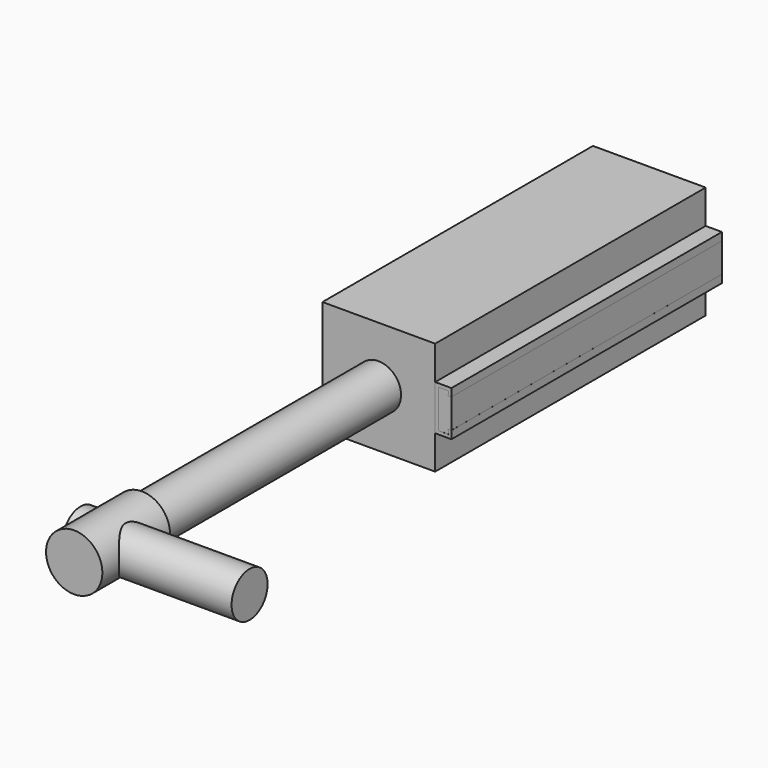
from build123d import *

# Parameters (mm, degrees)
F0_W              = 100
F0_H              = 300
F1_DEPTH          = 50
F2_R              = 20
F3_DEPTH          = 250
F4_DEPTH          = 300
F5_R              = 25
F6_DEPTH          = 37.5
F8_R              = 20
F9_DEPTH          = 50
F11_DEPTH         = 75
F18_D             = 3.5
F18_DEPTH         = 18
F18_CSINK_D       = 8.96
F18_CSINK_ANGLE   = 90
F18_TIP           = 1.0515060833
F18_2_D           = 3.5
F18_2_DEPTH       = 18
F18_2_CSINK_D     = 8.96
F18_2_CSINK_ANGLE = 90
F18_2_TIP         = 1.0515060833


# Not quite as in the source:
# - a feature of the source that left no trace in its solid (it failed there, or was rolled back) is left out


with BuildPart() as f1:
    # F0 (on Top) → F1 (new body, symmetric)
    with BuildSketch(Plane.XY):
        with Locations((0.3009543288, 62.5117615233)):
            Rectangle(F0_W, F0_H)
    extrude(amount=F1_DEPTH, both=True)

    # F2 (on face) → F3 (cut)
    with BuildSketch(Plane.XZ.offset(87.4882384767)):
        Circle(F2_R)
    extrude(amount=-F3_DEPTH, mode=Mode.SUBTRACT)

    # F18
    with Locations(Plane.YZ.offset(53.3009543288)):
        with Locations((162.5128239393, 0), (0, 0)):
            CounterSinkHole(F18_D / 2, F18_CSINK_D / 2, depth=F18_DEPTH, counter_sink_angle=F18_CSINK_ANGLE)
            with Locations((0, 0, -(F18_DEPTH + F18_TIP / 2))):  # 118° drill point
                Cone(0, F18_D / 2, F18_TIP, mode=Mode.SUBTRACT)


with BuildPart() as f4:
    # F2 (on face) → F4 (new body)
    with BuildSketch(Plane.XZ.offset(87.4882384767)):
        Circle(F2_R)
    extrude(amount=F4_DEPTH)

    # F5 (on face) → F6 (join, symmetric)
    with BuildSketch(Plane.XZ.offset(387.4882384767)):
        Circle(F5_R)
    extrude(amount=F6_DEPTH, both=True)


with BuildPart() as f9:
    # F8 (on Right) → F9 (new body, symmetric)
    with BuildSketch(Plane.YZ):
        with Locations((-386.7093552819, 0)):
            Circle(F8_R)
    extrude(amount=F9_DEPTH, both=True)


with BuildPart() as f4_1:
    add(f4.part)

    # F10: cut F9
    add(f9.part, mode=Mode.SUBTRACT)


with BuildPart() as f11:
    # F8 (on Right) → F11 (new body, symmetric)
    with BuildSketch(Plane.YZ):
        with Locations((-386.7093552819, 0)):
            Circle(F8_R)
    extrude(amount=F11_DEPTH, both=True)


with BuildPart() as f12_1:
    # F12: copy of F11
    add(f11.part.moved(Location((50, 0, 0))))


with BuildPart() as f16:
    # F16: sweep along a path in F15
    with BuildLine(Plane.YZ.offset(50.3009543288)) as f16_path:
        Line((-87.4882384767, 0), (212.5117615233, 0))
    # F14 (on face) → F16 (sweep)
    with BuildSketch(Plane(origin=(0, 212.5117615233, 0), x_dir=(-1, 0, 0), z_dir=(0, 1, 0))):
        Polygon((-50.3009543288, -20), (-50.3009543288, 20), (-64.7470878231, 20), (-64.7470878231, 13), (-61.7470878231, 13), (-62.3009543288, 16.9614684012), (-53.3009543288, 16.9614684012), (-53.3009543288, -17), (-62.3009543288, -17), (-61.7470878231, -13), (-64.7470878231, -13), (-64.7470878231, -20), align=None)
    sweep(path=f16_path.line)

    # F18#2
    with Locations(Plane.YZ.offset(53.3009543288)):
        with Locations((162.5128239393, 0), (0, 0)):
            CounterSinkHole(F18_2_D / 2, F18_2_CSINK_D / 2, depth=F18_2_DEPTH, counter_sink_angle=F18_2_CSINK_ANGLE)
            with Locations((0, 0, -(F18_2_DEPTH + F18_2_TIP / 2))):  # 118° drill point
                Cone(0, F18_2_D / 2, F18_2_TIP, mode=Mode.SUBTRACT)


with BuildPart() as f21:
    # F21: sweep along a path in F20
    with BuildLine(Plane.YZ.offset(53.3009543288)) as f21_path:
        Line((-87.4882384767, 0), (212.5117615233, -0.0192657994))
    # F19 (on face) → F21 (sweep)
    with BuildSketch(Plane(origin=(0, 212.5117615233, 0), x_dir=(-1, 0, 0), z_dir=(0, 1, 0))):
        Polygon((-61.7470878231, 13), (-64.7470878231, 13), (-64.7470878231, -13), (-61.7470878231, -13), (-62.3009543288, -17), (-53.3009543288, -17), (-53.3009543288, 16.9614684012), (-62.3009543288, 16.9614684012), align=None)
    sweep(path=f21_path.line)


solid = Compound([f1.part, f4_1.part, f12_1.part, f16.part, f21.part])
